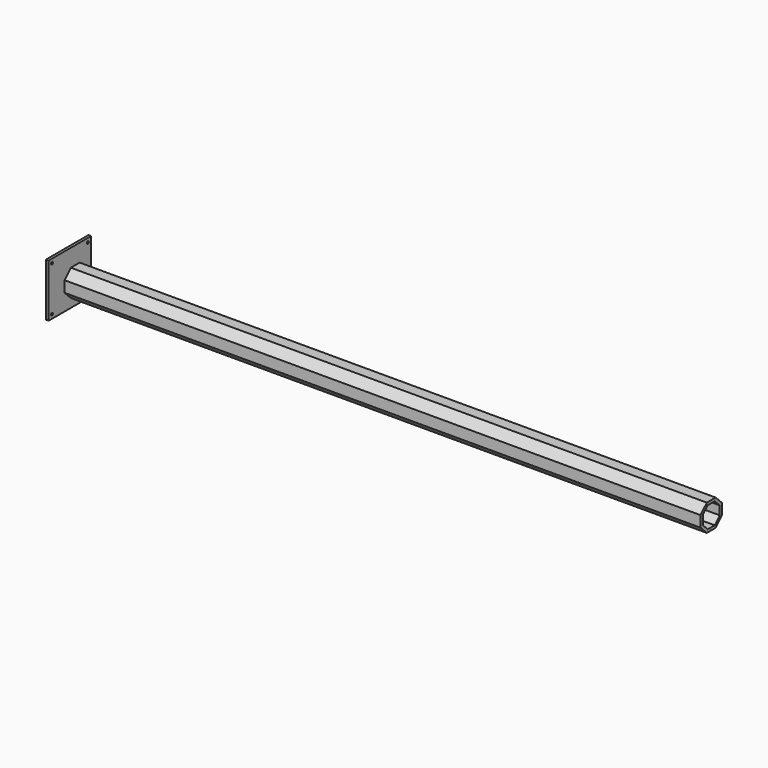
from build123d import *

# Parameters (mm, degrees)
F1_DEPTH = 762
F7_W     = 63.5
F7_H     = 63.5
F8_DEPTH = 3.175
F10_D    = 2.8448


# Not quite as in the source:
# - the program builds the solid bodies; features that only make, move or delete a surface that nothing else refers to are left out


with BuildPart() as f1:
    # F0 (on Right) → F1 (new body)
    with BuildSketch(Plane.YZ):
        Polygon((6.627416998, 16), (-6.627416998, 16), (-16, 6.627416998), (-16, -6.627416998), (-6.627416998, -16), (6.627416998, -16), (16, -6.627416998), (16, 6.627416998), align=None)
        Polygon((-12.7, 5.2605122421), (-5.2605122421, 12.7), (5.2605122421, 12.7), (12.7, 5.2605122421), (12.7, -5.2605122421), (5.2605122421, -12.7), (-5.2605122421, -12.7), (-12.7, -5.2605122421), align=None, mode=Mode.SUBTRACT)
    extrude(amount=F1_DEPTH)


with BuildPart() as f8:
    # F7 (on offset) → F8 (new body)
    with BuildSketch(Plane.YZ.offset(-6.35)):
        Rectangle(F7_W, F7_H)
    extrude(amount=-F8_DEPTH)

    # F10 (through all)
    with Locations(Plane.YZ.offset(-6.35)):
        with Locations((-26.924, 26.924), (26.924, 26.924), (26.924, -26.9015428433), (-26.924, -26.9010574487)):
            Hole(F10_D / 2)


solid = Compound([f1.part, f8.part])
